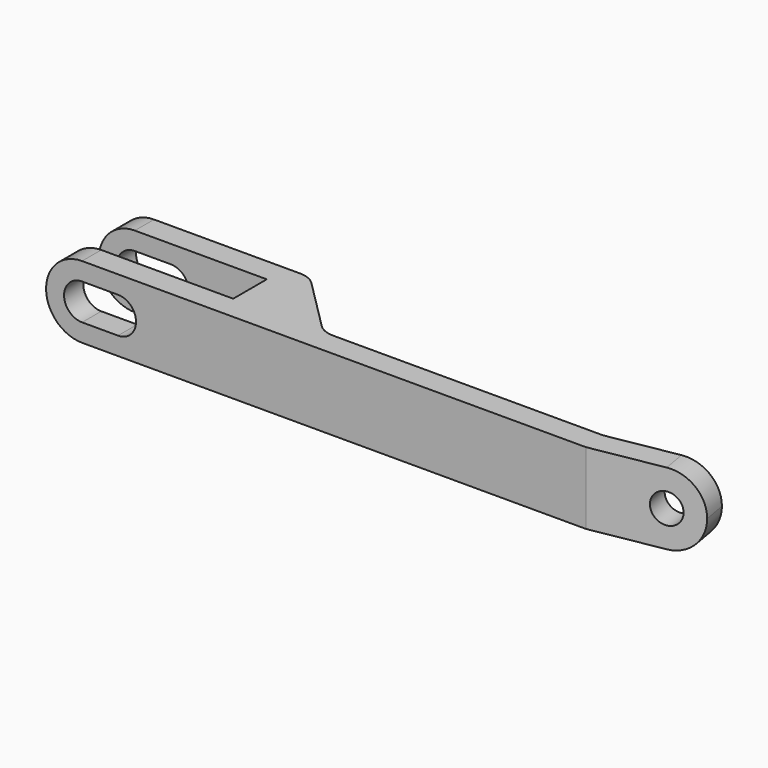
from build123d import *

# Parameters (mm, degrees)
F1_DEPTH = 6
F3_DEPTH = 25
F4_R     = 2.99999
F5_R     = 1.25
F6_DEPTH = 25
F7_R     = 2.99999


# Not quite as in the source:
# - a fillet or chamfer is up to 0.001 mm smaller than in the source, because OpenCascade refuses the exact size


with BuildPart() as f1:
    # F0 (on Top) → F1 (new body)
    with BuildSketch(Plane.XY):
        with BuildLine():
            Line((-22.5, -1), (22.5, -1))
            Line((22.5, -1), (31.3632697771, 0.562833599))
            Line((31.3632697771, 0.562833599), (31.0159734218, 2.532449105))
            Line((31.0159734218, 2.532449105), (22.3250226729, 1))
            Line((22.3250226729, 1), (-0.1715728753, 1))
            ThreePointArc((-0.1715728753, 1), (-0.93693974, 1.152240935), (-1.5857864376, 1.5857864376))
            Line((-1.5857864376, 1.5857864376), (-5.9142135624, 5.9142135624))
            ThreePointArc((-5.9142135624, 5.9142135624), (-6.56306026, 6.347759065), (-7.3284271247, 6.5))
            Line((-7.3284271247, 6.5), (-22.5, 6.5))
            Line((-22.5, 6.5), (-22.5, 4.5))
            Line((-22.5, 4.5), (-8.5, 4.5))
            Line((-8.5, 4.5), (-8.5, 1))
            Line((-8.5, 1), (-22.5, 1))
            Line((-22.5, 1), (-22.5, -1))
        make_face()
    extrude(amount=F1_DEPTH)

    # F2 (on face) → F3 (cut)
    with BuildSketch(Plane.XZ.offset(1)):
        with BuildLine():
            Line((-16.5, 4.5), (-19.5, 4.5))
            ThreePointArc((-19.5, 4.5), (-21, 2.999998177), (-19.499996354, 1.5))
            Line((-19.499996354, 1.5), (-16.5046735253, 1.5000072806))
            ThreePointArc((-16.5046735253, 1.5000072806), (-15.0000018202, 2.9976632345), (-16.5, 4.5))
        make_face()
    extrude(amount=-F3_DEPTH, mode=Mode.SUBTRACT)

    # F4 (radius 3 in the source; OpenCascade refuses exactly that, so slightly less here)
    f4_edges = [f1.edges().sort_by_distance(p)[0] for p in [
        (-22.5, 5.5, 6),
        (-22.5, 0, 6),
        (-22.5, 5.5, 0),
        (-22.5, 0, 0),
    ]]
    fillet(f4_edges, radius=F4_R)

    # F5 (on face) → F6 (cut)
    with BuildSketch(Plane(origin=(0.8494680878, -4.8175729228, 0), x_dir=(0.984807753, 0.1736481777, 0), z_dir=(0.1736481777, -0.984807753, 0))):
        with Locations((27.9845262651, 3)):
            Circle(F5_R)
    extrude(amount=-F6_DEPTH, mode=Mode.SUBTRACT)

    # F7 (radius 3 in the source; OpenCascade refuses exactly that, so slightly less here)
    f7_edges = [f1.edges().sort_by_distance(p)[0] for p in [
        (31.189622, 1.547641, 6),
        (31.189622, 1.547641, 0),
    ]]
    fillet(f7_edges, radius=F7_R)


solid = f1.part
